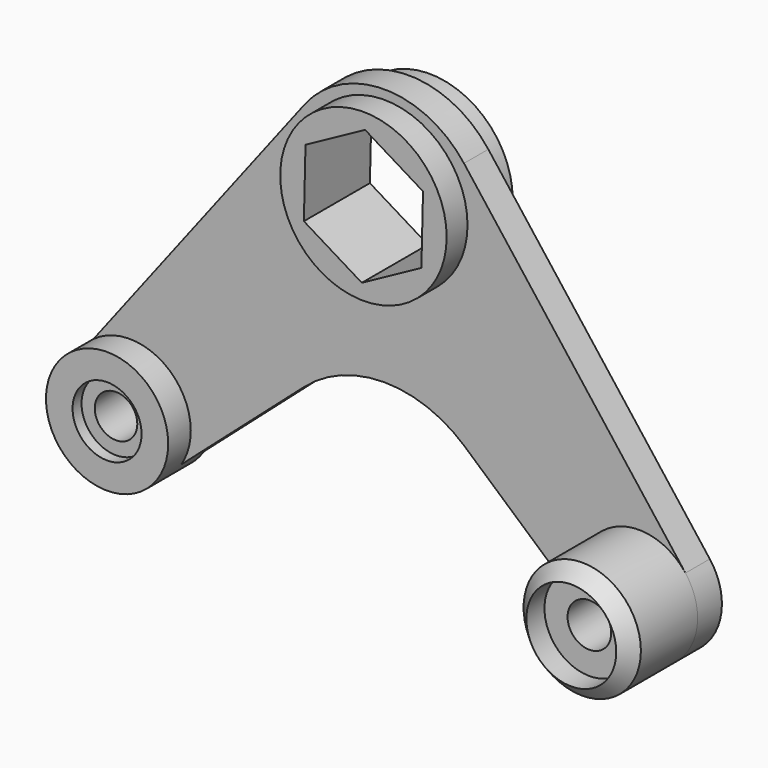
from build123d import *
from build123d import SkipClean  # not in build123d's __all__

# Parameters (mm, degrees)
F0_R      = 12.5377374601
F1_DEPTH  = 6.21636
F3_DEPTH  = 43.11412
F5_DEPTH  = 2.29052
F6_R      = 9.2054650922
F7_DEPTH  = 4.2521
F8_R      = 8.8363001854
F9_DEPTH  = 13.21401
F10_R     = 3.2055120306
F11_DEPTH = 28.79148
F12_R     = 5.1967625573
F13_DEPTH = 1.68604
F14_R     = 3.2868447942
F15_DEPTH = 33.07979
F16_R     = 6.7713245086
F17_DEPTH = 3.883
F20_DEPTH = 42.80702
F22_DEPTH = 12.5


# Not quite as in the source:
# - a fillet or chamfer that OpenCascade refuses, or shapes differently, is made with other operations: its cross-section is extruded or revolved along the edge and cut away or added
# - after a boolean that leaves OpenCascade's solid faulty, fix() repairs it


with BuildPart() as f1:
    # F0 (on Front) → F1 (new body, symmetric)
    with BuildSketch(Plane.XZ):
        Circle(F0_R)
    extrude(amount=F1_DEPTH, both=True)

    # F2 (on face) → F3 (cut)
    with BuildSketch(Plane.XZ.offset(6.21636)):
        Polygon((-1.5670347233, 8.3723281259), (-8.0341662075, 2.8290721839), (-6.4671314842, -5.5432559419), (1.5670347233, -8.3723281259), (8.0341662075, -2.8290721839), (6.4671314842, 5.5432559419), align=None)
    extrude(amount=-F3_DEPTH, mode=Mode.SUBTRACT)

    # F4 (on Front) → F5 (join, symmetric)
    with BuildSketch(Plane.XZ):
        with BuildLine():
            ThreePointArc((-32.5207371804, -47.4863935268), (-30.3092801317, -44.4938571079), (-29.5258178112, -40.8562750417))
            ThreePointArc((-29.5258178112, -40.8562750417), (-35.5217487699, -32.4889275753), (-45.3723830373, -35.4770199791))
            ThreePointArc((-45.3723830373, -35.4770199791), (-44.3951798921, -47.3124631688), (-32.5207371804, -47.4863935268))
        make_face()
        with BuildLine():
            ThreePointArc((-45.3723830373, -35.4770199791), (-35.5217487699, -32.4889275753), (-29.5258178112, -40.8562750417))
            ThreePointArc((-29.5258178112, -40.8562750417), (-30.3092801317, -44.4938571079), (-32.5207371804, -47.4863935268))
            Line((-32.5207371804, -47.4863935268), (-12.0985076262, -29.4936502279))
            ThreePointArc((-12.0985076262, -29.4936502279), (0, -24.9242672402), (12.0985076262, -29.4936502279))
            Line((12.0985076262, -29.4936502279), (32.5207371804, -47.4863935268))
            ThreePointArc((32.5207371804, -47.4863935268), (32.3290561012, -34.4000869145), (45.3723830373, -35.4770199791))
            Line((45.3723830373, -35.4770199791), (12.0060265403, 8.0061388902))
            ThreePointArc((12.0060265403, 8.0061388902), (0, 13.9267959918), (-12.0060265403, 8.0061388902))
            Line((-12.0060265403, 8.0061388902), (-45.3723830373, -35.4770199791))
        make_face()
        with BuildLine():
            ThreePointArc((47.1984181821, -40.8562750417), (46.729465463, -38.0159058149), (45.3723830373, -35.4770199791))
            ThreePointArc((45.3723830373, -35.4770199791), (32.3290561012, -34.4000869145), (32.5207371804, -47.4863935268))
            ThreePointArc((32.5207371804, -47.4863935268), (41.9997000629, -48.9091129066), (47.1984181821, -40.8562750417))
        make_face()
    extrude(amount=F5_DEPTH, both=True)

    # F6 (on face) → F7 (join, symmetric)
    with BuildSketch(Plane.XZ.offset(2.29052)):
        with Locations((-38.3621179966, -40.8562750417)):
            Circle(F6_R)
    extrude(amount=F7_DEPTH, both=True)

    # F8 (on face) → F9 (join)
    with BuildSketch(Plane.XZ.offset(2.29052)):
        with Locations((38.3621179966, -40.8562750417)):
            Circle(F8_R)
    with SkipClean():  # cleaning this boolean's faces spoils the solid; the shape is the same uncleaned
        extrude(amount=F9_DEPTH)

    # F10 (on face) → F11 (cut)
    with BuildSketch(Plane.XZ.offset(6.54262)):
        with Locations((-38.3621179966, -40.8562750417)):
            Circle(F10_R)
    extrude(amount=-F11_DEPTH, mode=Mode.SUBTRACT)

    add(f1.part.fix(), mode=Mode.REPLACE)

    # F12 (on face) → F13 (cut)
    with BuildSketch(Plane.XZ.offset(6.54262)):
        with Locations((-38.3621179966, -40.8562750417)):
            Circle(F12_R)
    extrude(amount=-F13_DEPTH, mode=Mode.SUBTRACT)

    # F14 (on face) → F15 (cut)
    with BuildSketch(Plane.XZ.offset(15.50453)):
        with Locations((38.3621179966, -40.8562750417)):
            Circle(F14_R)
    extrude(amount=-F15_DEPTH, mode=Mode.SUBTRACT)

    # F16 (on face) → F17 (cut)
    with BuildSketch(Plane.XZ.offset(15.50453)):
        with Locations((38.3621179966, -40.8562750417)):
            Circle(F16_R)
    extrude(amount=-F17_DEPTH, mode=Mode.SUBTRACT)

    # F18: chamfer of 2.54 on 1 edges, made by hand

    # F18_s1 → F18_t2 (revolve, cut)
    with BuildSketch(Plane.XY.offset(-40.8562750417)):
        Polygon((47.1984181821, -12.96453), (44.6584181821, -15.50453), (47.1984181821, -15.50453), align=None)
    revolve(axis=Axis((38.3621179966, -15.50453, -40.8562750417), (0, -1, 0)), mode=Mode.SUBTRACT)

    # F19 (on face) → F20 (cut)
    with BuildSketch(Plane.XZ.offset(2.29052)):
        Polygon((7.5046534745, -4.3328137037), (7.5046534745, 4.3328137037), (0, 8.6656274074), (-7.5046534745, 4.3328137037), (-7.5046534745, -4.3328137037), (0, -8.6656274074), align=None)
    extrude(amount=-F20_DEPTH, mode=Mode.SUBTRACT)

    # F21 (on Front) → F22 (cut, symmetric)
    with BuildSketch(Plane.XZ):
        Polygon((8.97537597, 4.8977579377), (0.2461051893, 10.2217825674), (-8.7292707806, 5.3240246297), (-8.97537597, -4.8977579377), (-0.2461051893, -10.2217825674), (8.7292707806, -5.3240246297), align=None)
    extrude(amount=F22_DEPTH, both=True, mode=Mode.SUBTRACT)


solid = f1.part
